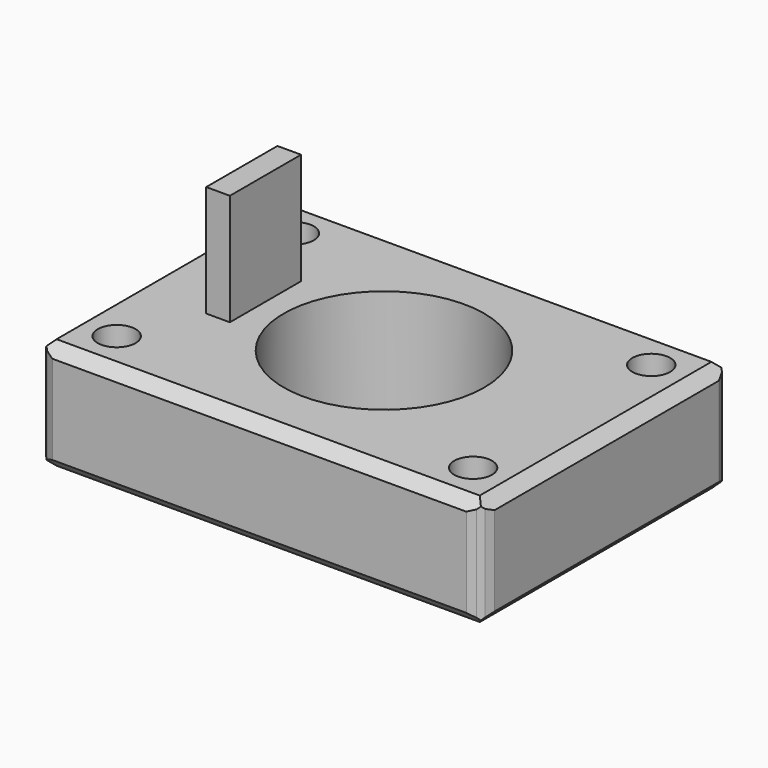
from build123d import *

# Parameters (mm, degrees)
F0_W        = 100
F0_H        = 70
F0_R        = 22.5
F1_DEPTH    = 25
F2_R        = 4.25
F3_DEPTH    = 25.001
F4_SIZE     = 2.5
F5_T1_DEPTH = 77.8584149398
F5_T3_DEPTH = 30.6428543011
F5_T5_DEPTH = 107.8584149398
F6_W        = 0.4621222615
F6_H        = 1.904300414
F7_DEPTH    = 25


# Not quite as in the source:
# - a fillet or chamfer that OpenCascade refuses, or shapes differently, is made with other operations: its cross-section is extruded or revolved along the edge and cut away or added


with BuildPart() as f1:
    # F0 (on Top) → F1 (new body)
    with BuildSketch(Plane.XY):
        Rectangle(F0_W, F0_H)
        Circle(F0_R, mode=Mode.SUBTRACT)
    extrude(amount=F1_DEPTH)

    # F2 (on face) → F3 (cut, through all)
    with BuildSketch(Plane.XY.offset(25)):
        with Locations((-40, 25)):
            Circle(F2_R)
        with Locations((-40, -25)):
            Circle(F2_R)
        with Locations((40, -25)):
            Circle(F2_R)
        with Locations((40, 25)):
            Circle(F2_R)
    extrude(amount=-F3_DEPTH, mode=Mode.SUBTRACT)

    # F4
    f4_edges = [f1.edges().sort_by_distance(p)[0] for p in [
        (50, 35, 12.5),
        (50, -35, 12.5),
        (-50, -35, 12.5),
        (-50, 35, 12.5),
    ]]
    chamfer(f4_edges, length=F4_SIZE)

    # F5: chamfer of 2.5 on 16 edges, made by hand

    # F5_s2 → F5_t1 (cut)
    with BuildSketch(Plane.XZ.offset(-38.9292074699)):
        Polygon((47.5, 25), (50, 22.5), (50, 25), align=None)
        Polygon((47.5, 0), (50, 2.5), (50, 0), align=None)
        Polygon((-47.5, 0), (-50, 2.5), (-50, 0), align=None)
        Polygon((-47.5, 25), (-50, 22.5), (-50, 25), align=None)
    extrude(amount=F5_T1_DEPTH, mode=Mode.SUBTRACT)

    # F5_s4 → F5_t3 (cut)
    with BuildSketch(Plane.XY.offset(-2.8214271505)):
        Polygon((49.267766953, -33.232233047), (50, -31.4644660941), (50, -32.5), align=None)
        Polygon((50, 31.4644660941), (49.267766953, 33.232233047), (50, 32.5), align=None)
        Polygon((-46.4644660941, -35), (-48.232233047, -34.267766953), (-47.5, -35), align=None)
        Polygon((46.4644660941, -35), (48.232233047, -34.267766953), (47.5, -35), align=None)
        Polygon((-50, 31.4644660941), (-49.267766953, 33.232233047), (-50, 32.5), align=None)
        Polygon((-49.267766953, -33.232233047), (-50, -31.4644660941), (-50, -32.5), align=None)
        Polygon((48.232233047, 34.267766953), (46.4644660941, 35), (47.5, 35), align=None)
        Polygon((-48.232233047, 34.267766953), (-46.4644660941, 35), (-47.5, 35), align=None)
    extrude(amount=F5_T3_DEPTH, mode=Mode.SUBTRACT)

    # F5_s6 → F5_t5 (cut)
    with BuildSketch(Plane.YZ.offset(-53.9292074699)):
        Polygon((-35, 2.5), (-32.5, 0), (-35, 0), align=None)
        Polygon((-35, 22.5), (-32.5, 25), (-35, 25), align=None)
        Polygon((32.5, 0), (35, 2.5), (35, 0), align=None)
        Polygon((32.5, 25), (35, 22.5), (35, 25), align=None)
    extrude(amount=F5_T5_DEPTH, mode=Mode.SUBTRACT)

    # F6 (on face) → F7 (join)
    with BuildSketch(Plane.XY.offset(25)):
        Polygon((-33.0991968513, 1.4772834256), (-33.0991968513, -8.5106156766), (-27.7881808579, -8.5106156766), (-27.7881808579, 11.4651825279), (-33.0991968513, 11.4651825279), (-33.0991968513, 3.3815838397), (-32.6370745897, 3.3815838397), (-32.6370745897, 1.4772834256), align=None)
        with Locations((-32.8681357205, 2.4294336326)):
            Rectangle(F6_W, F6_H)
    extrude(amount=F7_DEPTH)


solid = f1.part
